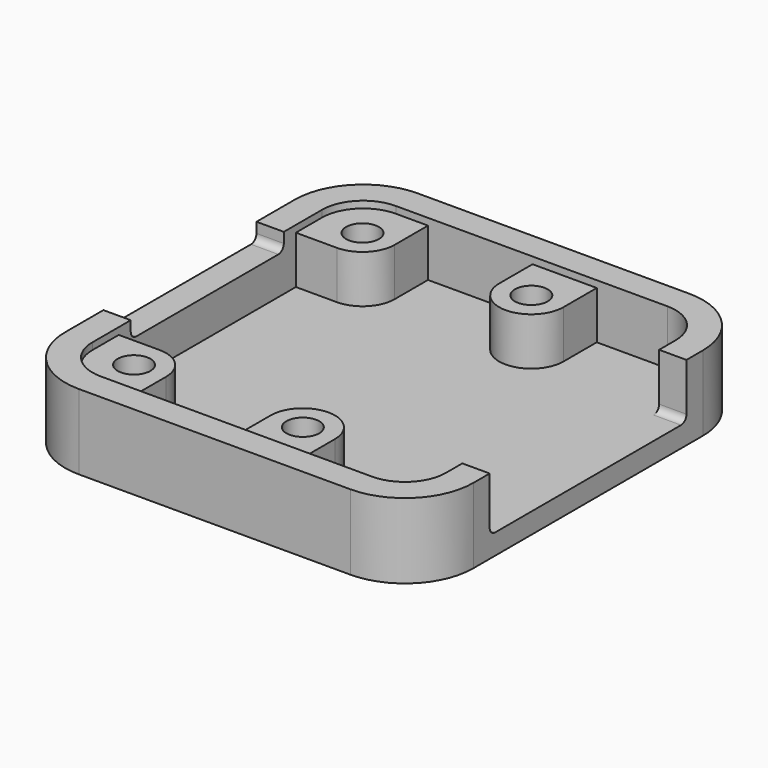
from build123d import *

# Parameters (mm, degrees)
F0_R     = 1.2
F1_DEPTH = 1.5
F2_DEPTH = 5
F3_DEPTH = 5.5
F5_DEPTH = 2
F7_DEPTH = 2


# Not quite as in the source:
# - a feature names something its author has since deleted; it is built from what else it names


with BuildPart() as f1:
    # F0 (on Top) → F1 (new body)
    with BuildSketch(Plane.XY):
        with BuildLine():
            Line((14.9310000289, -10.5), (14.9310000289, 10.5))
            ThreePointArc((14.9310000289, 10.5), (13.4665339264, 14.0355339264), (9.931, 15.5000000289))
            Line((9.931, 15.5000000289), (-9.931, 15.5000000289))
            ThreePointArc((-9.931, 15.5000000289), (-13.4665339264, 14.0355339264), (-14.9310000289, 10.5))
            Line((-14.9310000289, 10.5), (-14.9310000289, -10.5))
            ThreePointArc((-14.9310000289, -10.5), (-13.4665339264, -14.0355339264), (-9.931, -15.5000000289))
            Line((-9.931, -15.5000000289), (9.931, -15.5000000289))
            ThreePointArc((9.931, -15.5000000289), (13.4665339264, -14.0355339264), (14.9310000289, -10.5))
        make_face()
        with BuildLine():
            Line((-9.931, 13.5000000289), (-7.581, 13.5000000289))
            Line((-7.581, 13.5000000289), (0.069, 13.5000000289))
            Line((0.069, 13.5000000289), (4.769, 13.5000000289))
            Line((4.769, 13.5000000289), (9.931, 13.5000000289))
            ThreePointArc((9.931, 13.5000000289), (12.052320364, 12.621320364), (12.9310000289, 10.5))
            Line((12.9310000289, 10.5), (12.9310000289, -10.5))
            ThreePointArc((12.9310000289, -10.5), (12.052320364, -12.621320364), (9.931, -13.5000000289))
            Line((9.931, -13.5000000289), (4.769, -13.5000000289))
            Line((4.769, -13.5000000289), (0.069, -13.5000000289))
            Line((0.069, -13.5000000289), (-7.581, -13.5000000289))
            Line((-7.581, -13.5000000289), (-9.931, -13.5000000289))
            ThreePointArc((-9.931, -13.5000000289), (-12.052320364, -12.621320364), (-12.9310000289, -10.5))
            Line((-12.9310000289, -10.5), (-12.9310000289, -8.1))
            Line((-12.9310000289, -8.1), (-12.9310000289, 8.1))
            Line((-12.9310000289, 8.1), (-12.9310000289, 10.5))
            ThreePointArc((-12.9310000289, 10.5), (-12.052320364, 12.621320364), (-9.931, 13.5000000289))
        make_face(mode=Mode.SUBTRACT)
        with BuildLine():
            ThreePointArc((4.769, -10.45), (2.419, -8.1), (0.069, -10.45))
            ThreePointArc((0.069, -10.45), (2.419, -12.8), (4.769, -10.45))
        make_face()
        with Locations((2.419, -10.45)):
            Circle(F0_R, mode=Mode.SUBTRACT)
        with BuildLine():
            ThreePointArc((4.769, 10.45), (2.419, 12.8), (0.069, 10.45))
            ThreePointArc((0.069, 10.45), (2.419, 8.1), (4.769, 10.45))
        make_face()
        with Locations((2.419, 10.45)):
            Circle(F0_R, mode=Mode.SUBTRACT)
        with BuildLine():
            ThreePointArc((-9.931, 8.1), (-11.5927009358, 12.1117009358), (-7.581, 10.45))
            Line((-7.581, 10.45), (-7.581, 13.5000000289))
            Line((-7.581, 13.5000000289), (-9.931, 13.5000000289))
            ThreePointArc((-9.931, 13.5000000289), (-12.052320364, 12.621320364), (-12.9310000289, 10.5))
            Line((-12.9310000289, 10.5), (-12.9310000289, 8.1))
            Line((-12.9310000289, 8.1), (-9.931, 8.1))
        make_face()
        with BuildLine():
            Line((-9.931, -8.1), (-12.9310000289, -8.1))
            Line((-12.9310000289, -8.1), (-12.9310000289, -10.5))
            ThreePointArc((-12.9310000289, -10.5), (-12.052320364, -12.621320364), (-9.931, -13.5000000289))
            Line((-9.931, -13.5000000289), (-7.581, -13.5000000289))
            Line((-7.581, -13.5000000289), (-7.581, -10.45))
            ThreePointArc((-7.581, -10.45), (-11.5927009358, -12.1117009358), (-9.931, -8.1))
        make_face()
        with BuildLine():
            ThreePointArc((-7.581, -10.45), (-8.2692990642, -8.7882990642), (-9.931, -8.1))
            ThreePointArc((-9.931, -8.1), (-11.5927009358, -12.1117009358), (-7.581, -10.45))
        make_face()
        with Locations((-9.931, -10.45)):
            Circle(F0_R, mode=Mode.SUBTRACT)
        with BuildLine():
            Line((0.069, -10.45), (0.069, -13.5000000289))
            Line((0.069, -13.5000000289), (4.769, -13.5000000289))
            Line((4.769, -13.5000000289), (4.769, -10.45))
            ThreePointArc((4.769, -10.45), (2.419, -12.8), (0.069, -10.45))
        make_face()
        with BuildLine():
            ThreePointArc((-9.931, 8.1), (-8.2692990642, 8.7882990642), (-7.581, 10.45))
            ThreePointArc((-7.581, 10.45), (-11.5927009358, 12.1117009358), (-9.931, 8.1))
        make_face()
        with Locations((-9.931, 10.45)):
            Circle(F0_R, mode=Mode.SUBTRACT)
        with BuildLine():
            Line((4.769, 13.5000000289), (0.069, 13.5000000289))
            Line((0.069, 13.5000000289), (0.069, 10.45))
            ThreePointArc((0.069, 10.45), (2.419, 12.8), (4.769, 10.45))
            Line((4.769, 10.45), (4.769, 13.5000000289))
        make_face()
        with BuildLine():
            Line((-7.581, 13.5000000289), (-7.581, 10.45))
            ThreePointArc((-7.581, 10.45), (-8.2692990642, 8.7882990642), (-9.931, 8.1))
            Line((-9.931, 8.1), (-12.9310000289, 8.1))
            Line((-12.9310000289, 8.1), (-12.9310000289, -8.1))
            Line((-12.9310000289, -8.1), (-9.931, -8.1))
            ThreePointArc((-9.931, -8.1), (-8.2692990642, -8.7882990642), (-7.581, -10.45))
            Line((-7.581, -10.45), (-7.581, -13.5000000289))
            Line((-7.581, -13.5000000289), (0.069, -13.5000000289))
            Line((0.069, -13.5000000289), (0.069, -10.45))
            ThreePointArc((0.069, -10.45), (2.419, -8.1), (4.769, -10.45))
            Line((4.769, -10.45), (4.769, -13.5000000289))
            Line((4.769, -13.5000000289), (9.931, -13.5000000289))
            ThreePointArc((9.931, -13.5000000289), (12.052320364, -12.621320364), (12.9310000289, -10.5))
            Line((12.9310000289, -10.5), (12.9310000289, 10.5))
            ThreePointArc((12.9310000289, 10.5), (12.052320364, 12.621320364), (9.931, 13.5000000289))
            Line((9.931, 13.5000000289), (4.769, 13.5000000289))
            Line((4.769, 13.5000000289), (4.769, 10.45))
            ThreePointArc((4.769, 10.45), (2.419, 8.1), (0.069, 10.45))
            Line((0.069, 10.45), (0.069, 13.5000000289))
            Line((0.069, 13.5000000289), (-7.581, 13.5000000289))
        make_face()
    extrude(amount=F1_DEPTH)

    # F0 (on Top) → F2 (join)
    with BuildSketch(Plane.XY):
        with BuildLine():
            ThreePointArc((-9.931, 8.1), (-11.5927009358, 12.1117009358), (-7.581, 10.45))
            Line((-7.581, 10.45), (-7.581, 13.5000000289))
            Line((-7.581, 13.5000000289), (-9.931, 13.5000000289))
            ThreePointArc((-9.931, 13.5000000289), (-12.052320364, 12.621320364), (-12.9310000289, 10.5))
            Line((-12.9310000289, 10.5), (-12.9310000289, 8.1))
            Line((-12.9310000289, 8.1), (-9.931, 8.1))
        make_face()
        with BuildLine():
            ThreePointArc((-9.931, 8.1), (-8.2692990642, 8.7882990642), (-7.581, 10.45))
            ThreePointArc((-7.581, 10.45), (-11.5927009358, 12.1117009358), (-9.931, 8.1))
        make_face()
        with Locations((-9.931, 10.45)):
            Circle(F0_R, mode=Mode.SUBTRACT)
        with BuildLine():
            ThreePointArc((4.769, 10.45), (2.419, 12.8), (0.069, 10.45))
            ThreePointArc((0.069, 10.45), (2.419, 8.1), (4.769, 10.45))
        make_face()
        with Locations((2.419, 10.45)):
            Circle(F0_R, mode=Mode.SUBTRACT)
        with BuildLine():
            Line((4.769, 13.5000000289), (0.069, 13.5000000289))
            Line((0.069, 13.5000000289), (0.069, 10.45))
            ThreePointArc((0.069, 10.45), (2.419, 12.8), (4.769, 10.45))
            Line((4.769, 10.45), (4.769, 13.5000000289))
        make_face()
        with BuildLine():
            ThreePointArc((4.769, -10.45), (2.419, -8.1), (0.069, -10.45))
            ThreePointArc((0.069, -10.45), (2.419, -12.8), (4.769, -10.45))
        make_face()
        with Locations((2.419, -10.45)):
            Circle(F0_R, mode=Mode.SUBTRACT)
        with BuildLine():
            Line((0.069, -10.45), (0.069, -13.5000000289))
            Line((0.069, -13.5000000289), (4.769, -13.5000000289))
            Line((4.769, -13.5000000289), (4.769, -10.45))
            ThreePointArc((4.769, -10.45), (2.419, -12.8), (0.069, -10.45))
        make_face()
        with BuildLine():
            ThreePointArc((-7.581, -10.45), (-8.2692990642, -8.7882990642), (-9.931, -8.1))
            ThreePointArc((-9.931, -8.1), (-11.5927009358, -12.1117009358), (-7.581, -10.45))
        make_face()
        with Locations((-9.931, -10.45)):
            Circle(F0_R, mode=Mode.SUBTRACT)
        with BuildLine():
            Line((-9.931, -8.1), (-12.9310000289, -8.1))
            Line((-12.9310000289, -8.1), (-12.9310000289, -10.5))
            ThreePointArc((-12.9310000289, -10.5), (-12.052320364, -12.621320364), (-9.931, -13.5000000289))
            Line((-9.931, -13.5000000289), (-7.581, -13.5000000289))
            Line((-7.581, -13.5000000289), (-7.581, -10.45))
            ThreePointArc((-7.581, -10.45), (-11.5927009358, -12.1117009358), (-9.931, -8.1))
        make_face()
    extrude(amount=F2_DEPTH)

    # F0 (on Top) → F3 (join)
    with BuildSketch(Plane.XY):
        with BuildLine():
            Line((14.9310000289, -10.5), (14.9310000289, 10.5))
            ThreePointArc((14.9310000289, 10.5), (13.4665339264, 14.0355339264), (9.931, 15.5000000289))
            Line((9.931, 15.5000000289), (-9.931, 15.5000000289))
            ThreePointArc((-9.931, 15.5000000289), (-13.4665339264, 14.0355339264), (-14.9310000289, 10.5))
            Line((-14.9310000289, 10.5), (-14.9310000289, -10.5))
            ThreePointArc((-14.9310000289, -10.5), (-13.4665339264, -14.0355339264), (-9.931, -15.5000000289))
            Line((-9.931, -15.5000000289), (9.931, -15.5000000289))
            ThreePointArc((9.931, -15.5000000289), (13.4665339264, -14.0355339264), (14.9310000289, -10.5))
        make_face()
        with BuildLine():
            Line((-9.931, 13.5000000289), (-7.581, 13.5000000289))
            Line((-7.581, 13.5000000289), (0.069, 13.5000000289))
            Line((0.069, 13.5000000289), (4.769, 13.5000000289))
            Line((4.769, 13.5000000289), (9.931, 13.5000000289))
            ThreePointArc((9.931, 13.5000000289), (12.052320364, 12.621320364), (12.9310000289, 10.5))
            Line((12.9310000289, 10.5), (12.9310000289, -10.5))
            ThreePointArc((12.9310000289, -10.5), (12.052320364, -12.621320364), (9.931, -13.5000000289))
            Line((9.931, -13.5000000289), (4.769, -13.5000000289))
            Line((4.769, -13.5000000289), (0.069, -13.5000000289))
            Line((0.069, -13.5000000289), (-7.581, -13.5000000289))
            Line((-7.581, -13.5000000289), (-9.931, -13.5000000289))
            ThreePointArc((-9.931, -13.5000000289), (-12.052320364, -12.621320364), (-12.9310000289, -10.5))
            Line((-12.9310000289, -10.5), (-12.9310000289, -8.1))
            Line((-12.9310000289, -8.1), (-12.9310000289, 8.1))
            Line((-12.9310000289, 8.1), (-12.9310000289, 10.5))
            ThreePointArc((-12.9310000289, 10.5), (-12.052320364, 12.621320364), (-9.931, 13.5000000289))
        make_face(mode=Mode.SUBTRACT)
    extrude(amount=F3_DEPTH)

    # F4 (on face) → F5 (cut)
    with BuildSketch(Plane(origin=(-14.9310000289, 0, 0), x_dir=(0, -1, 0), z_dir=(-1, 0, 0))):
        with BuildLine():
            Line((7, 5.5), (-7, 5.5))
            Line((-7, 5.5), (-7, 4.75))
            ThreePointArc((-7, 4.75), (-6.8535533906, 4.3964466094), (-6.5, 4.25))
            Line((-6.5, 4.25), (6.5, 4.25))
            ThreePointArc((6.5, 4.25), (6.8535533906, 4.3964466094), (7, 4.75))
            Line((7, 4.75), (7, 5.5))
        make_face()
    extrude(amount=-F5_DEPTH, mode=Mode.SUBTRACT)

    # F6 (on face) → F7 (cut)
    with BuildSketch(Plane.YZ.offset(14.9310000289)):
        with BuildLine():
            Line((9, 2), (9, 5.5))
            Line((9, 5.5), (-9, 5.5))
            Line((-9, 5.5), (-9, 2))
            ThreePointArc((-9, 2), (-8.8535533906, 1.6464466094), (-8.5, 1.5))
            Line((-8.5, 1.5), (8.5, 1.5))
            ThreePointArc((8.5, 1.5), (8.8535533906, 1.6464466094), (9, 2))
        make_face()
    extrude(amount=-F7_DEPTH, mode=Mode.SUBTRACT)


solid = f1.part
